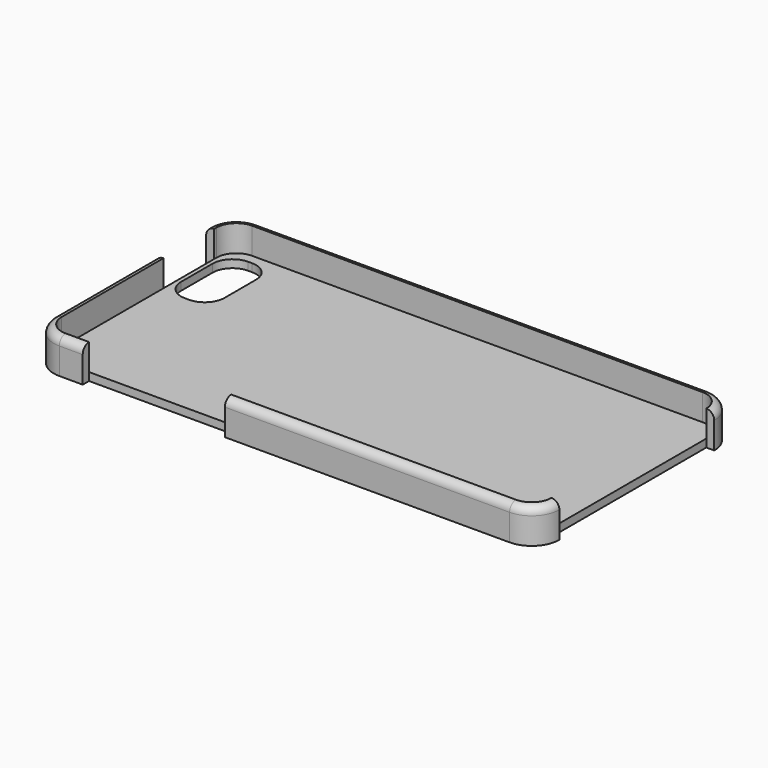
from build123d import *

# Parameters (mm, degrees)
F1_DEPTH = 2
F2_DEPTH = 8.7
F3_W     = 36
F3_H     = 8.7
F4_DEPTH = 2
F5_DEPTH = 2
F6_DEPTH = 2
F7_DEPTH = 2
F8_W     = 16
F8_H     = 8.7
F9_DEPTH = 2
F10_R    = 1.99999
F11_R    = 1.99999


# Not quite as in the source:
# - a fillet or chamfer is up to 0.001 mm smaller than in the source, because OpenCascade refuses the exact size


with BuildPart() as f1:
    # F0 (on Top) → F1 (new body)
    with BuildSketch(Plane.XY):
        with BuildLine():
            Line((57, 29.5), (-57, 29.5))
            ThreePointArc((-57, 29.5), (-60.5355339059, 28.0355339059), (-62, 24.5))
            Line((-62, 24.5), (-62, -24.5))
            ThreePointArc((-62, -24.5), (-60.5355339059, -28.0355339059), (-57, -29.5))
            Line((-57, -29.5), (57, -29.5))
            ThreePointArc((57, -29.5), (60.5355339059, -28.0355339059), (62, -24.5))
            Line((62, -24.5), (62, 24.5))
            ThreePointArc((62, 24.5), (60.5355339059, 28.0355339059), (57, 29.5))
        make_face()
        with BuildLine():
            Line((-56, 27.021933794), (-55, 27.021933794))
            ThreePointArc((-55, 27.021933794), (-51.4644660941, 25.5574677), (-50, 22.021933794))
            Line((-50, 22.021933794), (-50, 12.021933794))
            ThreePointArc((-50, 12.021933794), (-51.4644660941, 8.4863998881), (-55, 7.021933794))
            Line((-55, 7.021933794), (-56, 7.021933794))
            ThreePointArc((-56, 7.021933794), (-59.5355339059, 8.4863998881), (-61, 12.021933794))
            Line((-61, 12.021933794), (-61, 22.021933794))
            ThreePointArc((-61, 22.021933794), (-59.5355339059, 25.5574677), (-56, 27.021933794))
        make_face(mode=Mode.SUBTRACT)
    extrude(amount=F1_DEPTH)

    # F0 (on Top) → F2 (join)
    with BuildSketch(Plane.XY):
        with BuildLine():
            Line((57, 31.5), (-57, 31.5))
            ThreePointArc((-57, 31.5), (-61.9497474683, 29.4497474683), (-64, 24.5))
            Line((-64, 24.5), (-64, -24.5))
            ThreePointArc((-64, -24.5), (-61.9497474683, -29.4497474683), (-57, -31.5))
            Line((-57, -31.5), (57, -31.5))
            ThreePointArc((57, -31.5), (61.9497474683, -29.4497474683), (64, -24.5))
            Line((64, -24.5), (64, 24.5))
            ThreePointArc((64, 24.5), (61.9497474683, 29.4497474683), (57, 31.5))
        make_face()
        with BuildLine():
            ThreePointArc((-62, 24.5), (-60.5355339059, 28.0355339059), (-57, 29.5))
            Line((-57, 29.5), (57, 29.5))
            ThreePointArc((57, 29.5), (60.5355339059, 28.0355339059), (62, 24.5))
            Line((62, 24.5), (62, -24.5))
            ThreePointArc((62, -24.5), (60.5355339059, -28.0355339059), (57, -29.5))
            Line((57, -29.5), (-57, -29.5))
            ThreePointArc((-57, -29.5), (-60.5355339059, -28.0355339059), (-62, -24.5))
            Line((-62, -24.5), (-62, 24.5))
        make_face(mode=Mode.SUBTRACT)
    extrude(amount=F2_DEPTH)

    # F3 (on face) → F4 (cut)
    with BuildSketch(Plane.XZ.offset(31.5)):
        with Locations((-33.0772541165, 4.35)):
            Rectangle(F3_W, F3_H)
    extrude(amount=-F4_DEPTH, mode=Mode.SUBTRACT)

    # F5 (add): a face of the model
    f5_faces = [f1.faces().sort_by_distance(p)[0] for p in [
        (64, 0, 4.35),
    ]]
    extrude(f5_faces, amount=-F5_DEPTH)

    # F6 (add): a face of the model
    f6_faces = [f1.faces().sort_by_distance(p)[0] for p in [
        (64, 0, 4.35),
    ]]
    extrude(f6_faces, amount=-F6_DEPTH)

    # F7 (cut): a face of the model
    f7_faces = [f1.faces().sort_by_distance(p)[0] for p in [
        (64, 0, 4.35),
    ]]
    extrude(f7_faces, amount=-F7_DEPTH, mode=Mode.SUBTRACT)

    # F8 (on face) → F9 (cut)
    with BuildSketch(Plane(origin=(-64, 0, 0), x_dir=(0, -1, 0), z_dir=(-1, 0, 0))):
        with Locations((-15.7182565033, 4.35)):
            Rectangle(F8_W, F8_H)
    extrude(amount=-F9_DEPTH, mode=Mode.SUBTRACT)

    # F10 (radius 2 in the source; OpenCascade refuses exactly that, so slightly less here)
    f10_edges = [f1.edges().sort_by_distance(p)[0] for p in [
        (61.949747, 29.449747, 8.7),
        (0, 31.5, 8.7),
        (-61.949747, 29.449747, 8.7),
    ]]
    fillet(f10_edges, radius=F10_R)

    # F11 (radius 2 in the source; OpenCascade refuses exactly that, so slightly less here)
    f11_edges = [f1.edges().sort_by_distance(p)[0] for p in [
        (-64, -8.390872, 8.7),
        (-54.038627, -31.5, 8.7),
        (-61.949747, -29.449747, 8.7),
        (20.961373, -31.5, 8.7),
        (61.949747, -29.449747, 8.7),
    ]]
    fillet(f11_edges, radius=F11_R)


solid = f1.part
